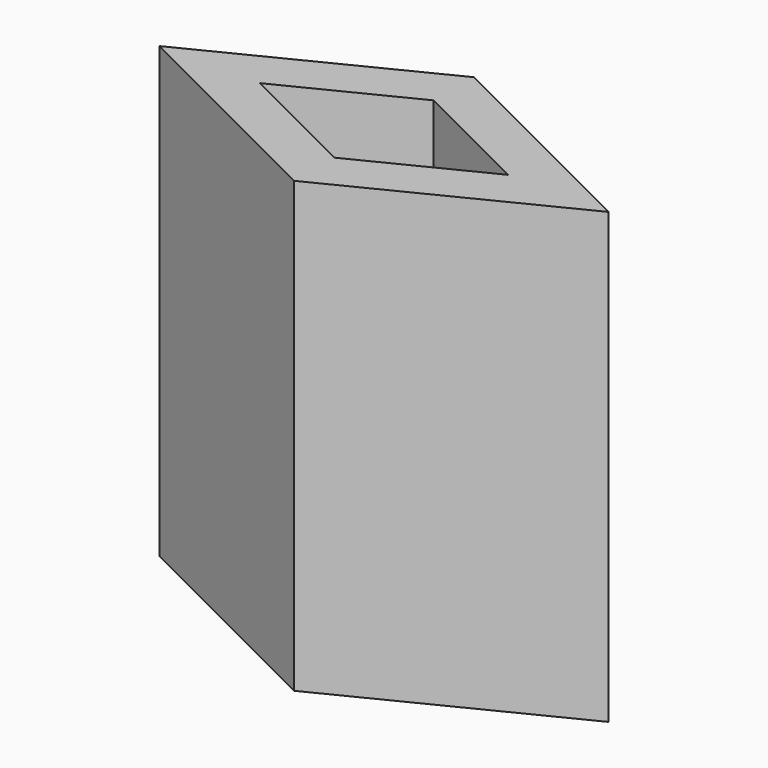
from build123d import *

# Parameters (mm, degrees)
F2_DEPTH = 5


# Not quite as in the source:
# - a pattern or mirror of a feature is missing from the dataset's text; its kind, count and spacing are read off the source's solid
# - a feature names something its author has since deleted; it is built from what else it names


with BuildPart() as f2:
    # F1 (on Top) → F2 (new body)
    with BuildSketch(Plane.XY):
        Polygon((0, 1.25), (0, 0.6909830056), (1.3819660113, 0), (2.5, 0), align=None)
    extrude(amount=F2_DEPTH)

    # F2_copies: F2 across plane


with BuildPart() as f2_1:
    add(f2.part)
    add(f2.part.mirror(Plane(origin=(0, 0, 0), x_dir=(0, 0, -1), z_dir=(0, -1, 0))))

    # F2_copies1: F2 across plane


with BuildPart() as f2_2:
    add(f2_1.part)
    add(f2_1.part.mirror(Plane(origin=(0, 0, 0), x_dir=(0, 0, -1), z_dir=(-1, 0, 0))))


solid = f2_2.part
